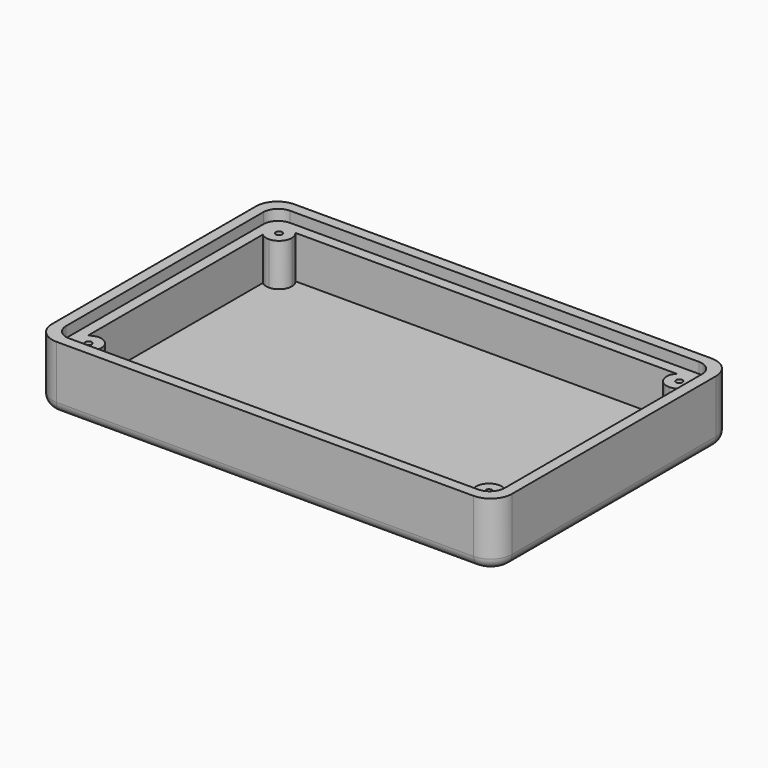
from build123d import *

# Parameters (mm, degrees)
F1_DEPTH  = 30
F2_T      = 10
F5_DEPTH  = 25
F7_W      = 195.9
F7_H      = 119.7
F8_DEPTH  = 5
F9_DEPTH  = 20
F10_D     = 3
F10_DEPTH = 10
F10_TIP   = 0.9012909285
F11_R     = 5


# Not quite as in the source:
# - a shell that OpenCascade refuses in one call is made with other operations: the cavity is built on its own and cut out


with BuildPart() as f1:
    # F0 (on Top) → F1 (new body)
    with BuildSketch(Plane.XY):
        with BuildLine():
            Line((-97.95, -69.85), (97.95, -69.85))
            ThreePointArc((97.95, -69.85), (105.0210678119, -66.9210678119), (107.95, -59.85))
            Line((107.95, -59.85), (107.95, 59.85))
            ThreePointArc((107.95, 59.85), (105.0210678119, 66.9210678119), (97.95, 69.85))
            Line((97.95, 69.85), (-97.95, 69.85))
            ThreePointArc((-97.95, 69.85), (-105.0210678119, 66.9210678119), (-107.95, 59.85))
            Line((-107.95, 59.85), (-107.95, -59.85))
            ThreePointArc((-107.95, -59.85), (-105.0210678119, -66.9210678119), (-97.95, -69.85))
        make_face()
    extrude(amount=F1_DEPTH)

    # F2: shell of thickness 10, made by hand


with BuildPart() as f2_core1:
    # F2_t2: copy of F1
    add(f1.part)

    # the walls: a layer under each face that stays
    f2_faces = [f2_core1.faces().sort_by_distance(p)[0] for p in [
        (0, -69.85, 15),
        (107.95, 0, 15),
        (0, 69.85, 15),
        (-107.95, 0, 15),
        (0, 0, 0),
    ]]
    thicken(f2_faces, amount=-F2_T, mode=Mode.SUBTRACT)


with BuildPart() as f1_1:
    add(f1.part)

    # what is left inside the walls is the cavity
    f2_cavity = [f2_core1.part.solids().sort_by_distance(p)[0] for p in [
        (0, -19.95, 10.1),
    ]]
    add(f2_cavity, mode=Mode.SUBTRACT)

    # F4 (on offset) → F5 (cut)
    with BuildSketch(Plane.XY.offset(25)):
        with BuildLine():
            Line((-95.95, -64.85), (95.95, -64.85))
            ThreePointArc((95.95, -64.85), (100.8997474683, -62.7997474683), (102.95, -57.85))
            Line((102.95, -57.85), (102.95, 57.85))
            ThreePointArc((102.95, 57.85), (100.8997474683, 62.7997474683), (95.95, 64.85))
            Line((95.95, 64.85), (-95.95, 64.85))
            ThreePointArc((-95.95, 64.85), (-100.8997474683, 62.7997474683), (-102.95, 57.85))
            Line((-102.95, 57.85), (-102.95, -57.85))
            ThreePointArc((-102.95, -57.85), (-100.8997474683, -62.7997474683), (-95.95, -64.85))
        make_face()
    extrude(amount=F5_DEPTH, mode=Mode.SUBTRACT)

    # F7 (on face) → F8 (cut)
    with BuildSketch(Plane.XY.offset(10)):
        Rectangle(F7_W, F7_H)
    extrude(amount=-F8_DEPTH, mode=Mode.SUBTRACT)

    # F6 (on face) → F9 (join, through all)
    with BuildSketch(Plane.XY.offset(25)):
        with BuildLine():
            Line((-93.95, 49.85), (-93.95, 55.85))
            Line((-93.95, 55.85), (-87.95, 55.85))
            ThreePointArc((-87.95, 55.85), (-88.3449658462, 57.9909325386), (-89.477864045, 59.85))
            Line((-89.477864045, 59.85), (-97.95, 59.85))
            Line((-97.95, 59.85), (-97.95, 51.377864045))
            ThreePointArc((-97.95, 51.377864045), (-96.0909325386, 50.2449658462), (-93.95, 49.85))
        make_face()
        with BuildLine():
            Line((-87.95, 55.85), (-93.95, 55.85))
            Line((-93.95, 55.85), (-93.95, 49.85))
            ThreePointArc((-93.95, 49.85), (-89.7073593129, 51.6073593129), (-87.95, 55.85))
        make_face()
        with BuildLine():
            Line((93.95, 55.85), (87.95, 55.85))
            ThreePointArc((87.95, 55.85), (89.7073593129, 51.6073593129), (93.95, 49.85))
            Line((93.95, 49.85), (93.95, 55.85))
        make_face()
        with BuildLine():
            ThreePointArc((89.477864045, 59.85), (88.3449658462, 57.9909325386), (87.95, 55.85))
            Line((87.95, 55.85), (93.95, 55.85))
            Line((93.95, 55.85), (93.95, 49.85))
            ThreePointArc((93.95, 49.85), (96.0909325386, 50.2449658462), (97.95, 51.377864045))
            Line((97.95, 51.377864045), (97.95, 59.85))
            Line((97.95, 59.85), (89.477864045, 59.85))
        make_face()
        with BuildLine():
            Line((93.95, -55.85), (93.95, -49.85))
            ThreePointArc((93.95, -49.85), (89.7073593129, -51.6073593129), (87.95, -55.85))
            Line((87.95, -55.85), (93.95, -55.85))
        make_face()
        with BuildLine():
            ThreePointArc((97.95, -51.377864045), (96.0909325386, -50.2449658462), (93.95, -49.85))
            Line((93.95, -49.85), (93.95, -55.85))
            Line((93.95, -55.85), (87.95, -55.85))
            ThreePointArc((87.95, -55.85), (88.3449658462, -57.9909325386), (89.477864045, -59.85))
            Line((89.477864045, -59.85), (97.95, -59.85))
            Line((97.95, -59.85), (97.95, -51.377864045))
        make_face()
        with BuildLine():
            Line((-93.95, -55.85), (-93.95, -49.85))
            ThreePointArc((-93.95, -49.85), (-96.0909325386, -50.2449658462), (-97.95, -51.377864045))
            Line((-97.95, -51.377864045), (-97.95, -59.85))
            Line((-97.95, -59.85), (-89.477864045, -59.85))
            ThreePointArc((-89.477864045, -59.85), (-88.3449658462, -57.9909325386), (-87.95, -55.85))
            Line((-87.95, -55.85), (-93.95, -55.85))
        make_face()
        with BuildLine():
            ThreePointArc((-87.95, -55.85), (-89.7073593129, -51.6073593129), (-93.95, -49.85))
            Line((-93.95, -49.85), (-93.95, -55.85))
            Line((-93.95, -55.85), (-87.95, -55.85))
        make_face()
    extrude(amount=-F9_DEPTH)

    # F10
    with Locations(Plane.XY.offset(25)):
        with Locations((-93.95, 55.85), (-93.95, -55.85), (93.95, -55.85), (93.95, 55.85)):
            Hole(F10_D / 2, depth=F10_DEPTH)
            with Locations((0, 0, -(F10_DEPTH + F10_TIP / 2))):  # 118° drill point
                Cone(0, F10_D / 2, F10_TIP, mode=Mode.SUBTRACT)

    # F11
    f11_edges = [f1_1.edges().sort_by_distance(p)[0] for p in [
        (-107.95, 0, 0),
    ]]
    fillet(f11_edges, radius=F11_R)


solid = f1_1.part
